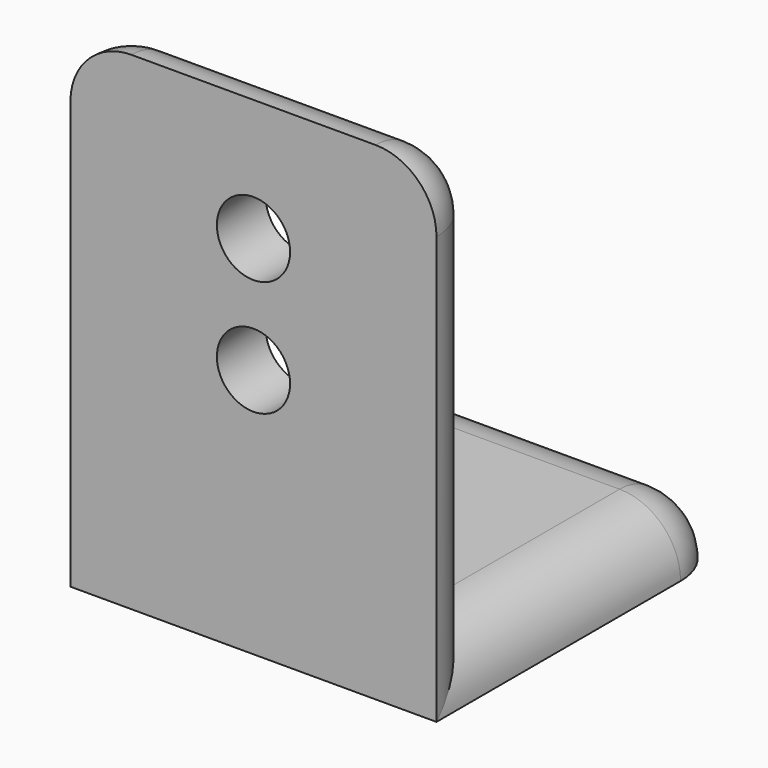
from build123d import *

# Parameters (mm, degrees)
F0_W     = 30
F0_H     = 30
F1_DEPTH = 5
F2_W     = 5
F2_H     = 35
F3_DEPTH = 30
F4_R     = 1.625
F5_DEPTH = 25
F6_R     = 4.99999
F7_R     = 3
F8_DEPTH = 25
F9_R     = 4.99999


# Not quite as in the source:
# - a fillet or chamfer is up to 0.001 mm smaller than in the source, because OpenCascade refuses the exact size


with BuildPart() as f1:
    # F0 (on Top) → F1 (new body)
    with BuildSketch(Plane.XY):
        with Locations((0, 15)):
            Rectangle(F0_W, F0_H)
    extrude(amount=F1_DEPTH)

    # F2 (on face) → F3 (join)
    with BuildSketch(Plane.YZ.offset(15)):
        with Locations((2.5, 22.5)):
            Rectangle(F2_W, F2_H)
    extrude(amount=-F3_DEPTH)

    # F4 (on face) → F5 (cut)
    with BuildSketch(Plane.XY.offset(5)):
        with Locations((0, 17.5)):
            Circle(F4_R)
    extrude(amount=-F5_DEPTH, mode=Mode.SUBTRACT)

    # F6 (radius 5 in the source; OpenCascade refuses exactly that, so slightly less here)
    f6_edges = [f1.edges().sort_by_distance(p)[0] for p in [
        (0, 30, 5),
        (15, 17.5, 5),
        (-15, 17.5, 5),
        (15, 30, 2.5),
        (-15, 30, 2.5),
    ]]
    fillet(f6_edges, radius=F6_R)

    # F7 (on face) → F8 (cut)
    with BuildSketch(Plane.XZ):
        with Locations((0, 30)):
            Circle(F7_R)
        with Locations((0, 20.5)):
            Circle(F7_R)
    extrude(amount=-F8_DEPTH, mode=Mode.SUBTRACT)

    # F9 (radius 5 in the source; OpenCascade refuses exactly that, so slightly less here)
    f9_edges = [f1.edges().sort_by_distance(p)[0] for p in [
        (15, 5, 20.000005),
        (-15, 5, 20.000005),
        (0, 5, 40),
        (15, 2.5, 40),
        (-15, 2.5, 40),
    ]]
    fillet(f9_edges, radius=F9_R)


solid = f1.part
